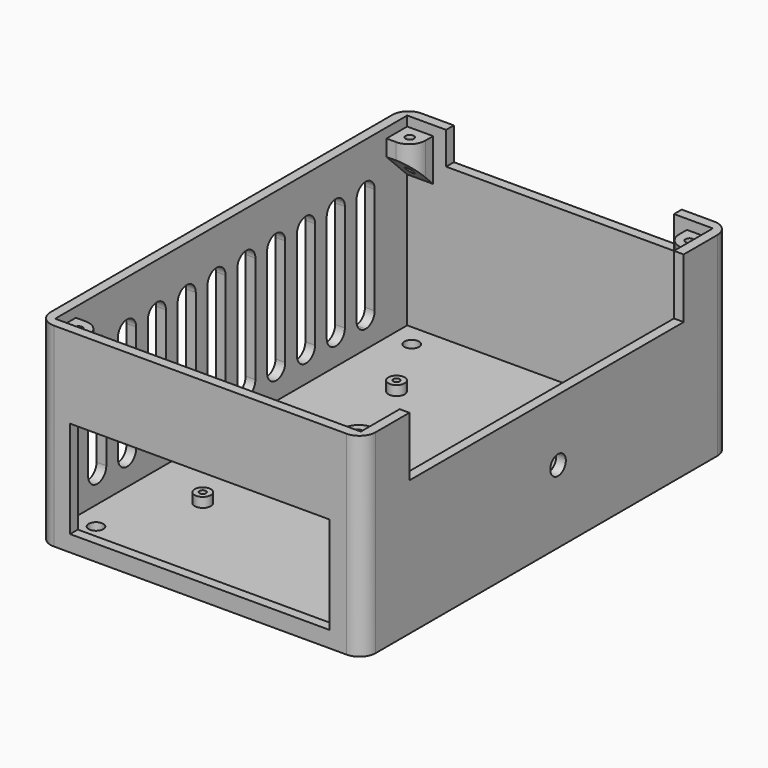
from build123d import *

# Parameters (mm, degrees)
F1_W           = 100.3
F1_H           = 141.77
F2_DEPTH       = 60
F3_T           = -3
F4_R           = 2
F5_DEPTH       = 25
F6_W           = 80
F6_H           = 30
F7_DEPTH       = 25
F8_W           = 105.77
F8_H           = 18.364803344
F9_DEPTH       = 25
F10_W          = 70.3
F10_H          = 10
F11_DEPTH      = 25
F12_R          = 2.25
F13_DEPTH      = 25
F15_DEPTH      = 8
F17_DEPTH      = 8
F19_R          = 1.25
F18_R          = 1.25
F20_R          = 1.25
F21_R          = 1.25
F22_DEPTH      = 25
F23_R          = 5
F24_R          = 5
F25_R          = 3
F26_DEPTH      = 25
F27_W          = 7
F27_H          = 40
F28_DEPTH      = 25
F29_R          = 3.49999
F31_DEPTH      = 25
F32_R          = 2.5
F32_R_2        = 1
F33_DEPTH      = 3
F33_DEPTH_BACK = 3


# Not quite as in the source:
# - a fillet or chamfer is up to 0.001 mm smaller than in the source, because OpenCascade refuses the exact size


with BuildPart() as f2:
    # F1 (on face) → F2 (new body)
    with BuildSketch(Plane.XY):
        with Locations((-6.5499655962, -8.0085539126)):
            Rectangle(F1_W, F1_H)
    extrude(amount=F2_DEPTH)

    # F3
    f3_openings = [f2.faces().sort_by_distance(p)[0] for p in [
        (-6.549966, -8.008554, 60),
    ]]
    offset(amount=F3_T, openings=f3_openings)

    # F4 (on face) → F5 (cut)
    with BuildSketch(Plane.XY.offset(3)):
        with Locations((-34.1999655962, 31.3764460874)):
            Circle(F4_R)
        with Locations((14.6000344038, 37.7764460874)):
            Circle(F4_R)
        with Locations((14.5000344038, -44.6235539126)):
            Circle(F4_R)
        with Locations((-34.1999655962, -43.3235539126)):
            Circle(F4_R)
    extrude(amount=-F5_DEPTH, mode=Mode.SUBTRACT)

    # F6 (on face) → F7 (cut)
    with BuildSketch(Plane.XZ.offset(78.8935539126)):
        with Locations((-6.6999655962, 20)):
            Rectangle(F6_W, F6_H)
    extrude(amount=-F7_DEPTH, mode=Mode.SUBTRACT)

    # F8 (on face) → F9 (cut)
    with BuildSketch(Plane.YZ.offset(43.6000344038)):
        with Locations((-8.0085539126, 50.817598328)):
            Rectangle(F8_W, F8_H)
    extrude(amount=-F9_DEPTH, mode=Mode.SUBTRACT)

    # F10 (on face) → F11 (cut)
    with BuildSketch(Plane(origin=(0, 62.8764460874, 0), x_dir=(-1, 0, 0), z_dir=(0, 1, 0))):
        with Locations((6.5499655962, 55)):
            Rectangle(F10_W, F10_H)
    extrude(amount=-F11_DEPTH, mode=Mode.SUBTRACT)

    # F12 (on face) → F13 (cut)
    with BuildSketch(Plane.XY.offset(3)):
        with Locations((-46.6999655962, 52.8764460874)):
            Circle(F12_R)
        with Locations((33.6000344038, 52.8764460874)):
            Circle(F12_R)
        with Locations((-46.6999655962, -68.8935539126)):
            Circle(F12_R)
    extrude(amount=-F13_DEPTH, mode=Mode.SUBTRACT)

    # F14 (on face) → F15 (join)
    with BuildSketch(Plane.YZ.offset(-53.6999655962)):
        Polygon((59.8764460874, 44), (59.8764460874, 57), (51.8764460874, 57), (51.8764460874, 52), align=None)
        Polygon((-75.8935539126, 57), (-75.8935539126, 44), (-67.8935539126, 52), (-67.8935539126, 57), align=None)
    extrude(amount=F15_DEPTH)

    # F16 (on face) → F17 (join)
    with BuildSketch(Plane(origin=(40.6000344038, 0, 0), x_dir=(0, -1, 0), z_dir=(-1, 0, 0))):
        Polygon((-59.8764460874, 57), (-59.8764460874, 44), (-51.8764460874, 52), (-51.8764460874, 57), align=None)
        Polygon((75.8935539126, 57), (67.8935539126, 57), (67.8935539126, 52), (75.8935539126, 44), align=None)
    extrude(amount=F17_DEPTH)

    # F19 (on face) + F18 (on face) + F20 (on face) + F21 (on face) → F22 (cut)
    with BuildSketch(Plane.XY.offset(57)):
        with Locations((-49.6999655962, 55.8764460874)):
            Circle(F19_R)
    with BuildSketch(Plane.XY.offset(57)):
        with Locations((36.6000344038, 55.8764460874)):
            Circle(F18_R)
    with BuildSketch(Plane.XY.offset(57)):
        with Locations((-49.6999655962, -71.8935539126)):
            Circle(F20_R)
    with BuildSketch(Plane.XY.offset(57)):
        with Locations((36.6000344038, -71.8935539126)):
            Circle(F21_R)
    extrude(amount=-F22_DEPTH, mode=Mode.SUBTRACT)

    # F23
    f23_edges = [f2.edges().sort_by_distance(p)[0] for p in [
        (-45.699966, 51.876446, 54.5),
        (32.600034, 51.876446, 54.5),
        (-45.699966, -67.893554, 54.5),
        (32.600034, -67.893554, 54.5),
    ]]
    fillet(f23_edges, radius=F23_R)

    # F24
    f24_edges = [f2.edges().sort_by_distance(p)[0] for p in [
        (43.600034, 62.876446, 30),
        (-56.699966, 62.876446, 30),
        (-56.699966, -78.893554, 30),
        (43.600034, -78.893554, 30),
    ]]
    fillet(f24_edges, radius=F24_R)

    # F25 (on face) → F26 (cut)
    with BuildSketch(Plane.YZ.offset(43.6000344038)):
        with Locations((-3.5735539126, 22.5)):
            Circle(F25_R)
    extrude(amount=-F26_DEPTH, mode=Mode.SUBTRACT)

    # F27 (on face) → F28 (cut)
    with BuildSketch(Plane(origin=(-56.6999655962, 0, 0), x_dir=(0, -1, 0), z_dir=(-1, 0, 0))):
        with Locations((-43.8384013922, 28.5368594155)):
            Rectangle(F27_W, F27_H)
    extrude(amount=-F28_DEPTH, mode=Mode.SUBTRACT)

    # F29 (radius 3.5 in the source; OpenCascade refuses exactly that, so slightly less here)
    f29_edges = [f2.edges().sort_by_distance(p)[0] for p in [
        (-55.199966, 40.338401, 48.536859),
        (-55.199966, 47.338401, 48.536859),
        (-55.199966, 40.338401, 8.536859),
        (-55.199966, 47.338401, 8.536859),
    ]]
    fillet(f29_edges, radius=F29_R)

    # F30 (on face) → F31 (cut)
    with BuildSketch(Plane(origin=(-56.6999655962, 0, 0), x_dir=(0, -1, 0), z_dir=(-1, 0, 0))):
        with BuildLine():
            Line((-40.3384013922, 12.0368594155), (-40.3384013922, 45.0368594155))
            ThreePointArc((-40.3384013922, 45.0368594155), (-43.8384013922, 48.5368594155), (-47.3384013922, 45.0368594155))
            Line((-47.3384013922, 45.0368594155), (-47.3384013922, 12.0368594155))
            ThreePointArc((-47.3384013922, 12.0368594155), (-43.8384013922, 8.5368594155), (-40.3384013922, 12.0368594155))
        make_face()
        with BuildLine():
            Line((-28.8384013922, 12.0368594155), (-28.8384013922, 45.0368594155))
            ThreePointArc((-28.8384013922, 45.0368594155), (-32.3384013922, 48.5368594155), (-35.8384013922, 45.0368594155))
            Line((-35.8384013922, 45.0368594155), (-35.8384013922, 12.0368594155))
            ThreePointArc((-35.8384013922, 12.0368594155), (-32.3384013922, 8.5368594155), (-28.8384013922, 12.0368594155))
        make_face()
        with BuildLine():
            Line((-17.3384013922, 12.0368594155), (-17.3384013922, 45.0368594155))
            ThreePointArc((-17.3384013922, 45.0368594155), (-20.8384013922, 48.5368594155), (-24.3384013922, 45.0368594155))
            Line((-24.3384013922, 45.0368594155), (-24.3384013922, 12.0368594155))
            ThreePointArc((-24.3384013922, 12.0368594155), (-20.8384013922, 8.5368594155), (-17.3384013922, 12.0368594155))
        make_face()
        with BuildLine():
            Line((-5.8384013922, 12.0368594155), (-5.8384013922, 45.0368594155))
            ThreePointArc((-5.8384013922, 45.0368594155), (-9.3384013922, 48.5368594155), (-12.8384013922, 45.0368594155))
            Line((-12.8384013922, 45.0368594155), (-12.8384013922, 12.0368594155))
            ThreePointArc((-12.8384013922, 12.0368594155), (-9.3384013922, 8.5368594155), (-5.8384013922, 12.0368594155))
        make_face()
        with BuildLine():
            Line((5.6615986078, 12.0368594155), (5.6615986078, 45.0368594155))
            ThreePointArc((5.6615986078, 45.0368594155), (2.1615986078, 48.5368594155), (-1.3384013922, 45.0368594155))
            Line((-1.3384013922, 45.0368594155), (-1.3384013922, 12.0368594155))
            ThreePointArc((-1.3384013922, 12.0368594155), (2.1615986078, 8.5368594155), (5.6615986078, 12.0368594155))
        make_face()
        with BuildLine():
            Line((17.1615986078, 12.0368594155), (17.1615986078, 45.0368594155))
            ThreePointArc((17.1615986078, 45.0368594155), (13.6615986078, 48.5368594155), (10.1615986078, 45.0368594155))
            Line((10.1615986078, 45.0368594155), (10.1615986078, 12.0368594155))
            ThreePointArc((10.1615986078, 12.0368594155), (13.6615986078, 8.5368594155), (17.1615986078, 12.0368594155))
        make_face()
        with BuildLine():
            Line((28.6615986078, 12.0368594155), (28.6615986078, 45.0368594155))
            ThreePointArc((28.6615986078, 45.0368594155), (25.1615986078, 48.5368594155), (21.6615986078, 45.0368594155))
            Line((21.6615986078, 45.0368594155), (21.6615986078, 12.0368594155))
            ThreePointArc((21.6615986078, 12.0368594155), (25.1615986078, 8.5368594155), (28.6615986078, 12.0368594155))
        make_face()
        with BuildLine():
            Line((40.1615986078, 12.0368594155), (40.1615986078, 45.0368594155))
            ThreePointArc((40.1615986078, 45.0368594155), (36.6615986078, 48.5368594155), (33.1615986078, 45.0368594155))
            Line((33.1615986078, 45.0368594155), (33.1615986078, 12.0368594155))
            ThreePointArc((33.1615986078, 12.0368594155), (36.6615986078, 8.5368594155), (40.1615986078, 12.0368594155))
        make_face()
        with BuildLine():
            Line((51.6615986078, 12.0368594155), (51.6615986078, 45.0368594155))
            ThreePointArc((51.6615986078, 45.0368594155), (48.1615986078, 48.5368594155), (44.6615986078, 45.0368594155))
            Line((44.6615986078, 45.0368594155), (44.6615986078, 12.0368594155))
            ThreePointArc((44.6615986078, 12.0368594155), (48.1615986078, 8.5368594155), (51.6615986078, 12.0368594155))
        make_face()
        with BuildLine():
            Line((63.1615986078, 12.0368594155), (63.1615986078, 45.0368594155))
            ThreePointArc((63.1615986078, 45.0368594155), (59.6615986078, 48.5368594155), (56.1615986078, 45.0368594155))
            Line((56.1615986078, 45.0368594155), (56.1615986078, 12.0368594155))
            ThreePointArc((56.1615986078, 12.0368594155), (59.6615986078, 8.5368594155), (63.1615986078, 12.0368594155))
        make_face()
    extrude(amount=-F31_DEPTH, mode=Mode.SUBTRACT)

    # F32 (on face) → F33 (join, two sides)
    with BuildSketch(Plane.XY.offset(3)) as f33_sk:
        with Locations((14.6000344038, 37.7764460874)):
            Circle(F32_R)
        with Locations((14.6000344038, 37.7764460874)):
            Circle(F32_R_2, mode=Mode.SUBTRACT)
        with Locations((14.5000344038, -44.6235539126)):
            Circle(F32_R)
        with Locations((14.5000344038, -44.6235539126)):
            Circle(F32_R_2, mode=Mode.SUBTRACT)
        with Locations((-34.1999655962, -43.3235539126)):
            Circle(F32_R)
        with Locations((-34.1999655962, -43.3235539126)):
            Circle(F32_R_2, mode=Mode.SUBTRACT)
        with Locations((-34.1999655962, 31.3764460874)):
            Circle(F32_R)
        with Locations((-34.1999655962, 31.3764460874)):
            Circle(F32_R_2, mode=Mode.SUBTRACT)
    extrude(amount=F33_DEPTH)
    extrude(f33_sk.sketch, amount=-F33_DEPTH_BACK)


solid = f2.part
